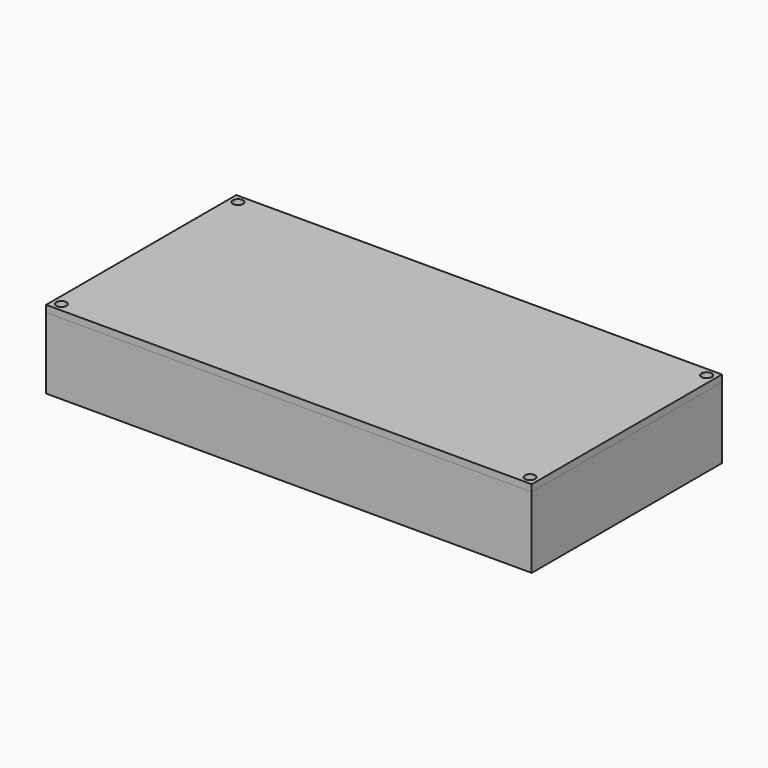
from build123d import *

# Parameters (mm, degrees)
F0_W     = 133
F0_H     = 60
F1_DEPTH = 8
F0_W_2   = 143
F0_H_2   = 70
F0_R     = 1.5
F2_DEPTH = 8.5
F3_W     = 143
F3_H     = 70
F3_W_2   = 129
F3_H_2   = 56
F4_DEPTH = 2
F5_DEPTH = 10.5
F6_W     = 133
F6_H     = 60
F7_DEPTH = 10.5
F8_W     = 143
F8_H     = 70
F8_R     = 1.5
F9_DEPTH = 2


# Not quite as in the source:
# - a feature names something its author has since deleted; it is built from what else it names


with BuildPart() as f1:
    # F0 (on Top) → F1 (new body)
    with BuildSketch(Plane.XY):
        with Locations((3.0246927018, 0)):
            Rectangle(F0_W, F0_H)
    extrude(amount=-F1_DEPTH)


with BuildPart() as f2:
    # F0 (on Top) → F2 (new body)
    with BuildSketch(Plane.XY):
        with Locations((3.0246927018, 0)):
            Rectangle(F0_W_2, F0_H_2)
        with Locations((-65.9753072982, -32.5)):
            Circle(F0_R, mode=Mode.SUBTRACT)
        with Locations((72.0246927018, -32.5)):
            Circle(F0_R, mode=Mode.SUBTRACT)
        with Locations((-65.9753072982, 32.5)):
            Circle(F0_R, mode=Mode.SUBTRACT)
        with Locations((3.0246927018, 0)):
            Rectangle(F0_W, F0_H, mode=Mode.SUBTRACT)
        with Locations((72.0246927018, 32.5)):
            Circle(F0_R, mode=Mode.SUBTRACT)
    extrude(amount=-F2_DEPTH)

    # F3 (on face) → F4 (join)
    with BuildSketch(Plane(origin=(0, 0, -8.5), x_dir=(1, 0, 0), z_dir=(0, 0, -1))):
        with Locations((3.0246927018, 0)):
            Rectangle(F3_W, F3_H)
        with Locations((3.0246927018, 0)):
            Rectangle(F3_W_2, F3_H_2, mode=Mode.SUBTRACT)
    extrude(amount=F4_DEPTH)

    # F0 (on Top) → F5 (join)
    with BuildSketch(Plane.XY):
        with Locations((3.0246927018, 0)):
            Rectangle(F0_W_2, F0_H_2)
        with Locations((-65.9753072982, -32.5)):
            Circle(F0_R, mode=Mode.SUBTRACT)
        with Locations((72.0246927018, -32.5)):
            Circle(F0_R, mode=Mode.SUBTRACT)
        with Locations((-65.9753072982, 32.5)):
            Circle(F0_R, mode=Mode.SUBTRACT)
        with Locations((3.0246927018, 0)):
            Rectangle(F0_W, F0_H, mode=Mode.SUBTRACT)
        with Locations((72.0246927018, 32.5)):
            Circle(F0_R, mode=Mode.SUBTRACT)
    extrude(amount=F5_DEPTH)

    # F6 (on face) → F7 (cut)
    with BuildSketch(Plane.XY.offset(10.5)):
        with BuildLine():
            ThreePointArc((-64.5610937358, 32), (-64.9146471264, 31.4393398282), (-65.4753072982, 31.0857864376))
            Line((-65.4753072982, 31.0857864376), (-65.4753072982, -31.0857864376))
            ThreePointArc((-65.4753072982, -31.0857864376), (-64.9146471264, -31.4393398282), (-64.5610937358, -32))
            Line((-64.5610937358, -32), (70.6104791395, -32))
            ThreePointArc((70.6104791395, -32), (70.9640325301, -31.4393398282), (71.5246927018, -31.0857864376))
            Line((71.5246927018, -31.0857864376), (71.5246927018, 31.0857864376))
            ThreePointArc((71.5246927018, 31.0857864376), (70.9640325301, 31.4393398282), (70.6104791395, 32))
            Line((70.6104791395, 32), (-64.5610937358, 32))
        make_face()
        with Locations((3.0246927018, 0)):
            Rectangle(F6_W, F6_H, mode=Mode.SUBTRACT)
    extrude(amount=-F7_DEPTH, mode=Mode.SUBTRACT)


with BuildPart() as f9:
    # F8 (on face) → F9 (new body)
    with BuildSketch(Plane.XY.offset(10.5)):
        with Locations((3.0246927018, 0)):
            Rectangle(F8_W, F8_H)
        with Locations((-65.9753072982, -32.5)):
            Circle(F8_R, mode=Mode.SUBTRACT)
        with Locations((72.0246927018, -32.5)):
            Circle(F8_R, mode=Mode.SUBTRACT)
        with Locations((-65.9753072982, 32.5)):
            Circle(F8_R, mode=Mode.SUBTRACT)
        with Locations((72.0246927018, 32.5)):
            Circle(F8_R, mode=Mode.SUBTRACT)
    extrude(amount=F9_DEPTH)


solid = Compound([f1.part, f2.part, f9.part])
